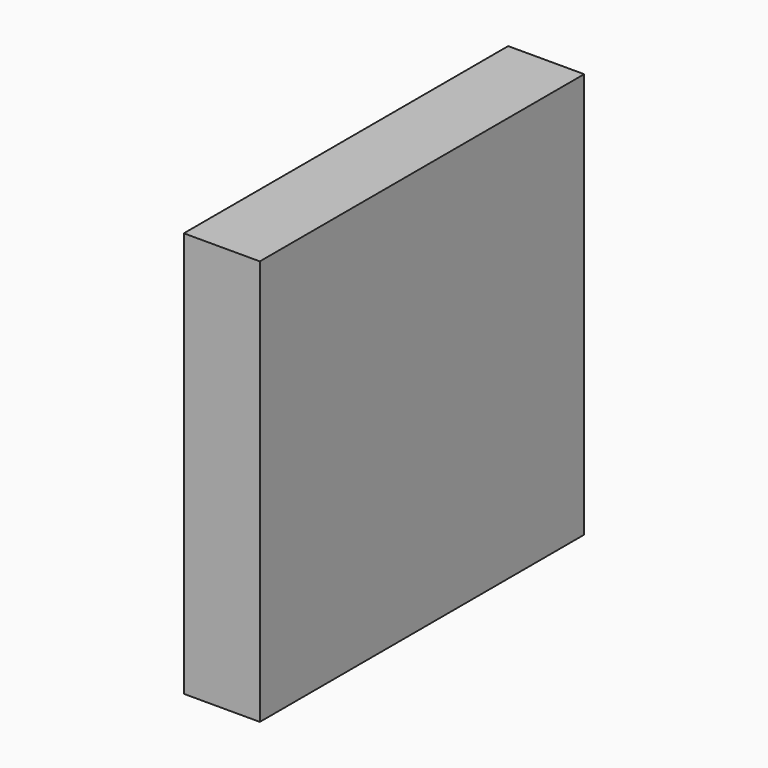
from build123d import *

# Parameters (mm, degrees)
F0_W     = 50.8
F0_H     = 50.8
F1_DEPTH = 9.525


# Not quite as in the source:
# - a length typed as a fraction of an inch, garbled in the dataset ("3 / 203.2 mm" for 3/8 in), is restored


with BuildPart() as f1:
    # F0 (on Right) → F1 (new body)
    with BuildSketch(Plane.YZ):
        Rectangle(F0_W, F0_H)
    extrude(amount=F1_DEPTH)


solid = f1.part
